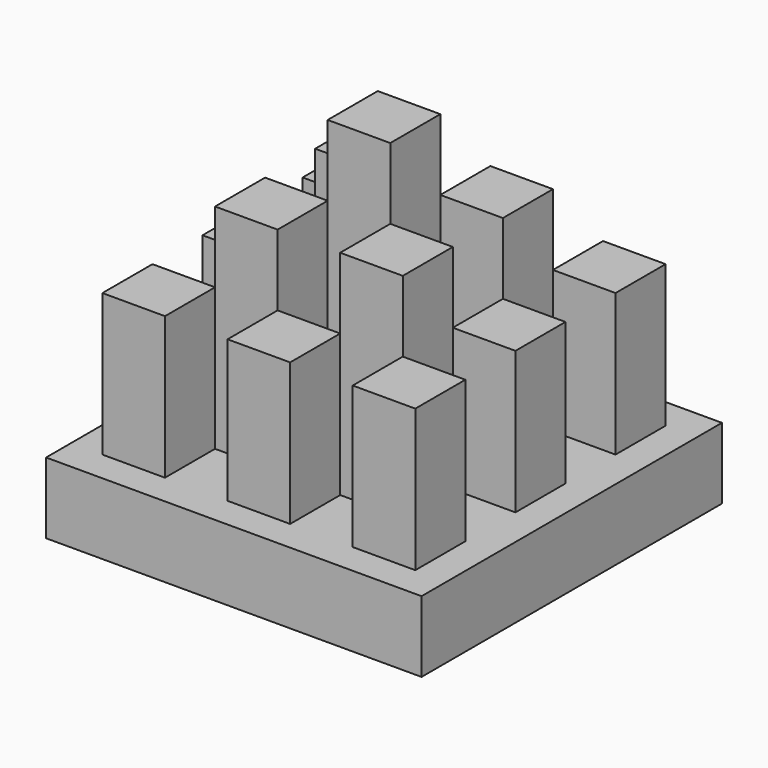
from build123d import *

# Parameters (mm, degrees)
F0_W     = 44
F0_H     = 44
F1_DEPTH = 100
F0_W_2   = 264
F0_H_2   = 264
F4_DEPTH = 50
F5_W     = 44
F5_H     = 44
F6_DEPTH = 150
F7_DEPTH = 100


# Not quite as in the source:
# - a feature names something its author has since deleted; it is built from what else it names


with BuildPart() as f1:
    # F0 (on Top) → F1 (new body)
    with BuildSketch(Plane.XY):
        with Locations((-88, 0)):
            Rectangle(F0_W, F0_H)
    extrude(amount=F1_DEPTH)


with BuildPart() as f1b:
    # F0 (on Top) → F1, piece 2 (new body)
    with BuildSketch(Plane.XY):
        with Locations((-88, 88)):
            Rectangle(F0_W, F0_H)
    extrude(amount=F1_DEPTH)


with BuildPart() as f1c:
    # F0 (on Top) → F1, piece 3 (new body)
    with BuildSketch(Plane.XY):
        with Locations((0, 88)):
            Rectangle(F0_W, F0_H)
    extrude(amount=F1_DEPTH)


with BuildPart() as f1d:
    # F0 (on Top) → F1, piece 4 (new body)
    with BuildSketch(Plane.XY):
        Rectangle(F0_W, F0_H)
    extrude(amount=F1_DEPTH)


with BuildPart() as f2_1:
    # F2: instance of F1
    add(f1.part.mirror(Plane.YZ))


with BuildPart() as f2_2:
    # F2: instance of F1b
    add(f1b.part.mirror(Plane.YZ))


with BuildPart() as f3_1:
    # F3: instance of F1b
    add(f1b.part.mirror(Plane.XZ))


with BuildPart() as f3_2:
    # F3: instance of F1c
    add(f1c.part.mirror(Plane.XZ))


with BuildPart() as f3_3:
    # F3: instance of F2_2
    add(f2_2.part.mirror(Plane.XZ))


with BuildPart() as f1_1:
    add(f1.part)

    add(f1b.part)  # F4 merges F1b

    add(f1c.part)  # F4 merges F1c

    add(f1d.part)  # F4 merges F1d

    add(f2_1.part)  # F4 merges F2_1

    add(f2_2.part)  # F4 merges F2_2

    add(f3_1.part)  # F4 merges F3_1

    add(f3_2.part)  # F4 merges F3_2

    add(f3_3.part)  # F4 merges F3_3
    # F0 (on Top) → F4 (join)
    with BuildSketch(Plane.XY):
        Rectangle(F0_W_2, F0_H_2)
        with Locations((-88, 0)):
            Rectangle(F0_W, F0_H, mode=Mode.SUBTRACT)
        with Locations((-88, 88)):
            Rectangle(F0_W, F0_H, mode=Mode.SUBTRACT)
        Rectangle(F0_W, F0_H, mode=Mode.SUBTRACT)
        with Locations((0, 88)):
            Rectangle(F0_W, F0_H, mode=Mode.SUBTRACT)
        with Locations((-88, 0)):
            Rectangle(F0_W, F0_H)
        Rectangle(F0_W, F0_H)
        with Locations((-88, 88)):
            Rectangle(F0_W, F0_H)
        with Locations((0, 88)):
            Rectangle(F0_W, F0_H)
    extrude(amount=-F4_DEPTH)

    # F7 (add): a face of the model
    f7_faces = [f1_1.faces().sort_by_distance(p)[0] for p in [
        (0, 0, 100),
    ]]
    extrude(f7_faces, amount=F7_DEPTH)


with BuildPart() as f6:
    # F5 (on face) → F6 (new body)
    with BuildSketch(Plane.XY):
        with Locations((-44, 44)):
            Rectangle(F5_W, F5_H)
    extrude(amount=F6_DEPTH)


with BuildPart() as f6b:
    # F5 (on face) → F6, piece 2 (new body)
    with BuildSketch(Plane.XY):
        with Locations((44, 44)):
            Rectangle(F5_W, F5_H)
    extrude(amount=F6_DEPTH)


with BuildPart() as f6c:
    # F5 (on face) → F6, piece 3 (new body)
    with BuildSketch(Plane.XY):
        with Locations((44, -44)):
            Rectangle(F5_W, F5_H)
    extrude(amount=F6_DEPTH)


with BuildPart() as f6d:
    # F5 (on face) → F6, piece 4 (new body)
    with BuildSketch(Plane.XY):
        with Locations((-44, -44)):
            Rectangle(F5_W, F5_H)
    extrude(amount=F6_DEPTH)


solid = Compound([f1_1.part, f6.part, f6b.part, f6c.part, f6d.part])
